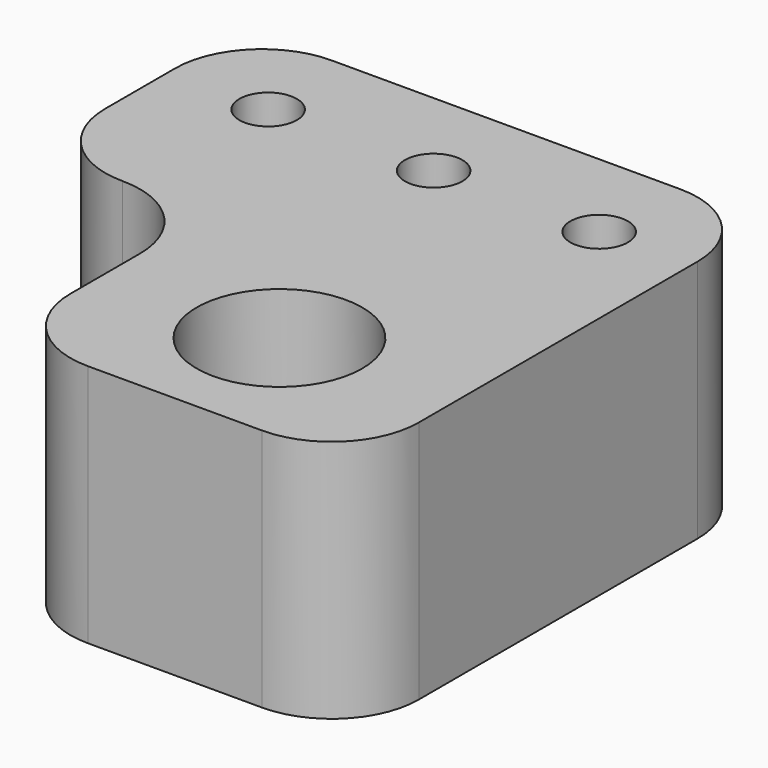
from build123d import *

# Parameters (mm, degrees)
F0_W      = 20
F0_H      = 30
F1_DEPTH  = 14
F2_R      = 2.65
F3_DEPTH  = 14.001
F4_R      = 1.65
F5_DEPTH  = 14.001
F6_W      = 15
F6_H      = 14
F7_DEPTH  = 10
F8_R      = 1.65
F9_DEPTH  = 14.001
F10_R     = 4.99999
F12_DEPTH = 8
F13_R     = 4.75
F14_DEPTH = 10


# Not quite as in the source:
# - a fillet or chamfer is up to 0.001 mm smaller than in the source, because OpenCascade refuses the exact size


with BuildPart() as f1:
    # F0 (on Top) → F1 (new body)
    with BuildSketch(Plane.XY):
        Rectangle(F0_W, F0_H)
    extrude(amount=F1_DEPTH)

    # F2 (on face) → F3 (cut, through all)
    with BuildSketch(Plane.XY.offset(14)):
        with Locations((0, -7.5)):
            Circle(F2_R)
    extrude(amount=-F3_DEPTH, mode=Mode.SUBTRACT)

    # F4 (on face) → F5 (cut, through all)
    with BuildSketch(Plane.XY.offset(14)):
        with Locations((-4.75, 9.5)):
            Circle(F4_R)
        with Locations((4.75, 9.5)):
            Circle(F4_R)
    extrude(amount=-F5_DEPTH, mode=Mode.SUBTRACT)

    # F6 (on face) → F7 (join)
    with BuildSketch(Plane(origin=(-10, 0, 0), x_dir=(0, -1, 0), z_dir=(-1, 0, 0))):
        with Locations((-7.5, 7)):
            Rectangle(F6_W, F6_H)
    extrude(amount=F7_DEPTH)

    # F8 (on face) → F9 (cut, through all)
    with BuildSketch(Plane.XY.offset(14)):
        with Locations((-14.25, 9.5)):
            Circle(F8_R)
    extrude(amount=-F9_DEPTH, mode=Mode.SUBTRACT)

    # F10 (radius 5 in the source; OpenCascade refuses exactly that, so slightly less here)
    f10_edges = [f1.edges().sort_by_distance(p)[0] for p in [
        (-12.6, 9.5, 7),
        (-10, -15, 7),
        (10, -15, 7),
        (-10, 0, 7),
        (-20, 0, 7),
        (-20, 15, 7),
        (10, 15, 7),
    ]]
    fillet(f10_edges, radius=F10_R)

    # F11 (on face) → F12 (cut)
    with BuildSketch(Plane(origin=(0, 0, 0), x_dir=(1, 0, 0), z_dir=(0, 0, -1))):
        Polygon((-17.5697640478, -9.5), (-15.9098820239, -12.375), (-12.5901179761, -12.375), (-10.9302359522, -9.5), (-12.5901179761, -6.625), (-15.9098820239, -6.625), align=None)
        Polygon((3.0901179761, -6.625), (1.4302359522, -9.5), (3.0901179761, -12.375), (6.4098820239, -12.375), (8.0697640478, -9.5), (6.4098820239, -6.625), align=None)
        Polygon((-6.4098820239, -6.625), (-8.0697640478, -9.5), (-6.4098820239, -12.375), (-3.0901179761, -12.375), (-1.4302359522, -9.5), (-3.0901179761, -6.625), align=None)
    extrude(amount=-F12_DEPTH, mode=Mode.SUBTRACT)

    # F13 (on face) → F14 (cut)
    with BuildSketch(Plane.XY.offset(14)):
        with Locations((0, -7.5)):
            Circle(F13_R)
    extrude(amount=-F14_DEPTH, mode=Mode.SUBTRACT)


solid = f1.part
